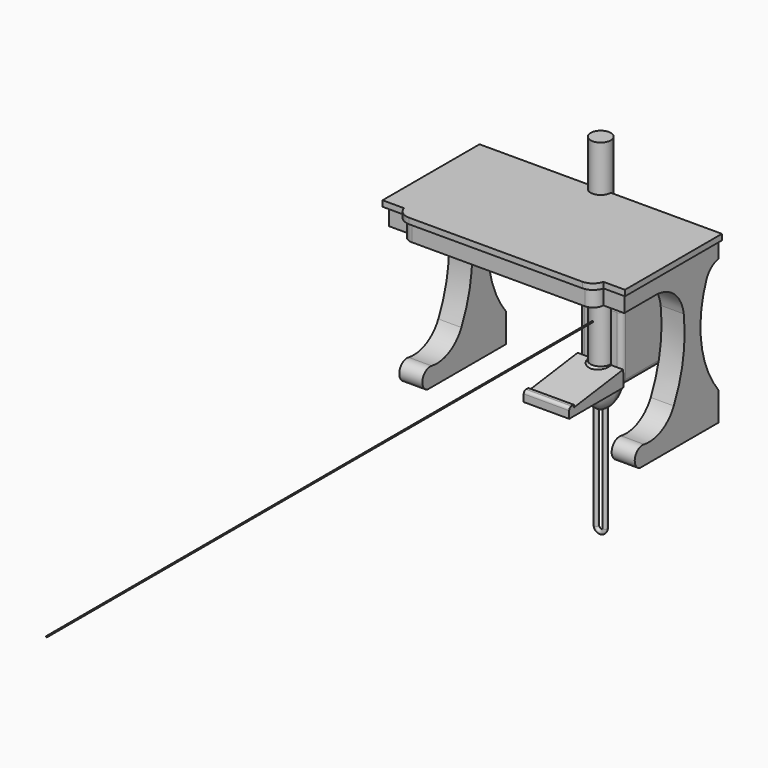
from build123d import *

# Parameters (mm, degrees)
F5_START       = 711.2
F5_DEPTH       = 25.4
F7_DEPTH       = 711.2
F9_DEPTH       = 533.401
F9_DEPTH_BACK  = 533.401
F10_W          = 833.12
F10_H          = 635
F11_DEPTH      = 577.851
F14_W          = 200.66
F14_H          = 282.7608090788
F14_W_2        = 149.86
F14_H_2        = 231.9608090788
F15_DEPTH      = 76.2
F16_W          = 184.15
F16_H          = 254
F17_DEPTH      = 301.625
F20_R          = 20.32
F23_DEPTH      = 100.0125
F25_DEPTH      = 100.0125
F26_R          = 44.45
F27_DEPTH      = 939.8
F28_R          = 9.525
F21_R          = 2.54
F31_DEPTH      = 3048
F31_DEPTH_BACK = 25.4


# Not quite as in the source:
# - the program builds the solid bodies; features that only make, move or delete a surface that nothing else refers to are left out


with BuildPart() as f5:
    # F4 (on Top) → F5 (new body)
    with BuildSketch(Plane.XY.offset(F5_START)):
        with BuildLine():
            Line((-533.4, 0), (-533.4, -533.4))
            Line((-533.4, -533.4), (-438.9283678228, -533.4))
            ThreePointArc((-438.9283678228, -533.4), (-417.5085548146, -565.4570155832), (-381, -577.85))
            Line((-381, -577.85), (381, -577.85))
            ThreePointArc((381, -577.85), (417.5085548146, -565.4570155832), (438.9283678228, -533.4))
            Line((438.9283678228, -533.4), (533.4, -533.4))
            Line((533.4, -533.4), (533.4, 0))
            Line((533.4, 0), (-533.4, 0))
        make_face()
    extrude(amount=F5_DEPTH)

    # F6 (on face) → F7 (join, through all)
    with BuildSketch(Plane(origin=(0, 0, 711.2), x_dir=(1, 0, 0), z_dir=(0, 0, -1))):
        with BuildLine():
            Line((-518.16, 518.16), (-518.16, 0))
            Line((-518.16, 0), (518.16, 0))
            Line((518.16, 0), (518.16, 518.16))
            Line((518.16, 518.16), (425.7309713578, 518.16))
            ThreePointArc((425.7309713578, 518.16), (412.5303912861, 549.6078375751), (381, 562.61))
            Line((381, 562.61), (-381, 562.61))
            ThreePointArc((-381, 562.61), (-412.5303912861, 549.6078375751), (-425.7309713578, 518.16))
            Line((-425.7309713578, 518.16), (-518.16, 518.16))
        make_face()
    extrude(amount=F7_DEPTH)

    # F8 (on Right) → F9 (cut, two sides)
    with BuildSketch(Plane.YZ) as f9_sk:
        with BuildLine():
            Line((-345.9380314084, 635), (-562.61, 635))
            Line((-562.61, 635), (-562.61, 0))
            Line((-562.61, 0), (-434.3815147877, 0))
            ThreePointArc((-434.3815147877, 0), (-458.6931603156, 52.4582878797), (-409.2337833345, 82.4032057154))
            ThreePointArc((-409.2337833345, 82.4032057154), (-313.5988706318, 95.8682445626), (-245.7028764243, 164.552142016))
            ThreePointArc((-245.7028764243, 164.552142016), (-193.7783043744, 327.7204304067), (-190.9851431847, 498.9286363125))
            ThreePointArc((-190.9851431847, 498.9286363125), (-242.8290919504, 596.1536279319), (-345.9380314084, 635))
        make_face()
        with BuildLine():
            Line((0, 126.2527257204), (0, 635))
            ThreePointArc((0, 635), (-39.8308571438, 616.8139248726), (-65.8426731825, 581.5915465355))
            ThreePointArc((-65.8426731825, 581.5915465355), (-94.2815076438, 345.0493638003), (0, 126.2527257204))
        make_face()
    extrude(amount=-F9_DEPTH, mode=Mode.SUBTRACT)
    extrude(f9_sk.sketch, amount=F9_DEPTH_BACK, mode=Mode.SUBTRACT)

    # F10 (on Front) → F11 (cut, through all)
    with BuildSketch(Plane.XZ):
        with Locations((0, 317.5)):
            Rectangle(F10_W, F10_H)
    extrude(amount=F11_DEPTH, mode=Mode.SUBTRACT)


with BuildPart() as f13:
    # F12 (on Front) → F13 (revolve)
    with BuildSketch(Plane.XZ):
        with BuildLine():
            Line((0, -115.9804045394), (0, 87.2195954606))
            add(Edge.make_bspline(
                [(0, 87.2195954606), (-7.5118135216, 87.2195954606), (-83.1378174289, 76.2777922663), (-82.1298262727, -76.7930781948), (-6.3140622444, -115.9804045394), (0, -115.9804045394)],
                knots=[0, 0, 0, 0, 0.2804581269, 0.6921777603, 1, 1, 1, 1], degree=3))
        make_face()
    revolve(axis=Axis((0, 0, -14.3804045394), (0, 0, -1)))

    # F14 (on Front) → F15 (cut, symmetric)
    with BuildSketch(Plane.XZ):
        Rectangle(F14_W, F14_H)
        Rectangle(F14_W_2, F14_H_2, mode=Mode.SUBTRACT)
    extrude(amount=F15_DEPTH, both=True, mode=Mode.SUBTRACT)


with BuildPart() as f17:
    # F16 (on Top) → F17 (new body)
    with BuildSketch(Plane.XY):
        with Locations((0, 127)):
            Rectangle(F16_W, F16_H)
    extrude(amount=F17_DEPTH)

    # F18 (on Right) → F19 (revolve, cut)
    with BuildSketch(Plane.YZ):
        with BuildLine():
            ThreePointArc((3.81, 228.6), (0.9730178895, 234.6704053668), (0, 241.3))
            Line((0, 241.3), (-2.54, 241.3))
            Line((-2.54, 241.3), (-2.54, 220.6397045256))
            Line((-2.54, 220.6397045256), (0, 220.6397045256))
            ThreePointArc((0, 220.6397045256), (0.1730968025, 221.9545052747), (0.6805909488, 223.1797045256))
            Line((0.6805909488, 223.1797045256), (3.81, 228.6))
        make_face()
    revolve(axis=Axis((0, 11.5358333333, 241.3), (0, 1, 0)), mode=Mode.SUBTRACT)

    # F20
    f20_edges = [f17.edges().sort_by_distance(p)[0] for p in [
        (92.075, 127, 301.625),
        (-92.075, 127, 301.625),
        (-92.075, 127, 0),
        (92.075, 127, 0),
        (0, 0, 0),
        (92.075, 0, 150.8125),
        (-92.075, 0, 150.8125),
        (0, 0, 301.625),
    ]]
    fillet(f20_edges, radius=F20_R)

    # F21 (on face) → F31 (join, two sides)
    with BuildSketch(Plane.XZ) as f31_sk:
        with Locations((0, 241.3)):
            Circle(F21_R)
    extrude(amount=F31_DEPTH)
    extrude(f31_sk.sketch, amount=-F31_DEPTH_BACK)


with BuildPart() as f23:
    # F22 (on Right) → F23 (new body, symmetric)
    with BuildSketch(Plane.YZ):
        with BuildLine():
            Line((0, 0), (0, 46.0375))
            Line((0, 46.0375), (-273.05, 26.9875))
            Line((-273.05, 26.9875), (-273.05, 44.45))
            Line((-273.05, 44.45), (-285.75, 44.45))
            ThreePointArc((-285.75, 44.45), (-294.7302561211, 40.7302561211), (-298.45, 31.75))
            Line((-298.45, 31.75), (-298.45, 0))
            Line((-298.45, 0), (0, 0))
        make_face()
    extrude(amount=F23_DEPTH, both=True)


with BuildPart() as f25:
    # F24 (on Right) → F25 (new body, symmetric)
    with BuildSketch(Plane.YZ):
        with BuildLine():
            Line((0, 0), (0, 46.0375))
            Line((0, 46.0375), (-0.2201697476, 46.0221393199))
            Line((-0.2201697476, 46.0221393199), (-1.9327220028, 70.5687216449))
            Line((-1.9327220028, 70.5687216449), (-273.05, 33.3529355393))
            Line((-273.05, 33.3529355393), (-273.05, 44.45))
            Line((-273.05, 44.45), (-285.75, 44.45))
            ThreePointArc((-285.75, 44.45), (-294.7302561211, 40.7302561211), (-298.45, 31.75))
            Line((-298.45, 31.75), (-298.45, 0))
            Line((-298.45, 0), (0, 0))
        make_face()
    extrude(amount=F25_DEPTH, both=True)


with BuildPart() as f27:
    # F26 (on Top) → F27 (new body)
    with BuildSketch(Plane.XY):
        Circle(F26_R)
    extrude(amount=F27_DEPTH)


with BuildPart() as f30:
    # F30: sweep along a path in F29
    with BuildLine(Plane.XZ) as f30_path:
        ThreePointArc((19.05, -19.05), (0, 0), (-19.05, -19.05))
        Line((-19.05, -19.05), (-19.05, -571.5))
        ThreePointArc((-19.05, -571.5), (0, -590.55), (19.05, -571.5))
        Line((19.05, -571.5), (19.05, -19.05))
    # F28 (on Right) → F30 (sweep)
    with BuildSketch(Plane.YZ):
        Circle(F28_R)
    sweep(path=f30_path.line)


solid = Compound([f5.part, f13.part, f17.part, f23.part, f25.part, f27.part, f30.part])
